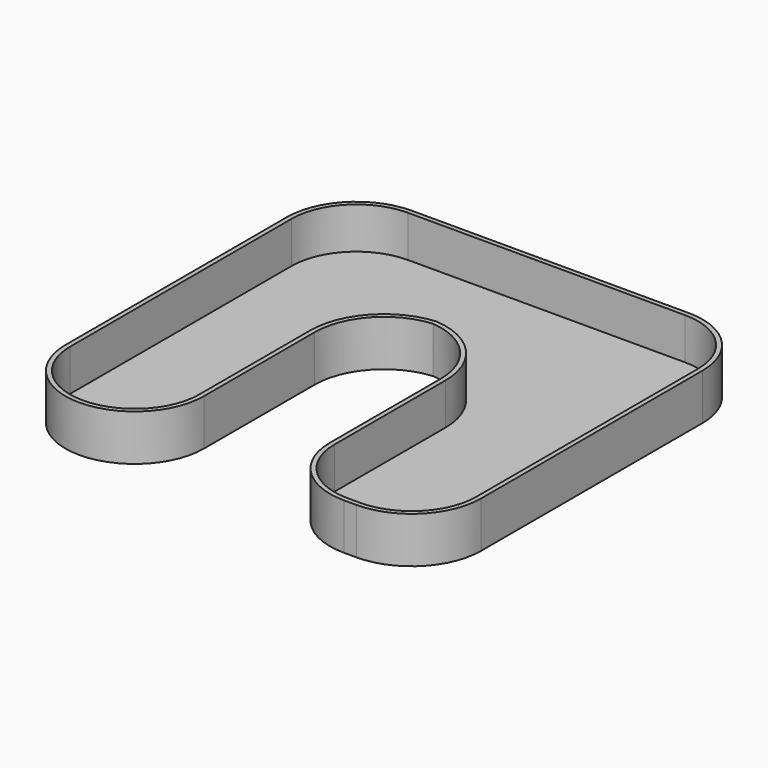
from build123d import *

# Parameters (mm, degrees)
F1_DEPTH    = 10
F2_T1_DEPTH = 10
F2_T3_DEPTH = 85
F3_T        = -1


# Not quite as in the source:
# - a fillet or chamfer that OpenCascade refuses, or shapes differently, is made with other operations: its cross-section is extruded or revolved along the edge and cut away or added


with BuildPart() as f1:
    # F0 (on Top) → F1 (new body)
    with BuildSketch(Plane.XY):
        Polygon((0, 90), (0, 0), (30, 0), (30, 60), (57.2968044168, 60), (57.2968044168, 0), (90, 0), (90, 90), align=None)
    extrude(amount=F1_DEPTH)

    # F2: fillet of radius 15 on 8 edges, made by hand

    # F2_s2 → F2_t1 (join)
    with BuildSketch(Plane.XY):
        with BuildLine():
            ThreePointArc((42.2968044168, 60), (52.9034061346, 55.6066017178), (57.2968044168, 45))
            Line((57.2968044168, 45), (57.2968044168, 60))
            Line((57.2968044168, 60), (42.2968044168, 60))
        make_face()
        with BuildLine():
            ThreePointArc((30, 45), (34.3933982822, 55.6066017178), (45, 60))
            Line((45, 60), (30, 60))
            Line((30, 60), (30, 45))
        make_face()
    extrude(amount=F2_T1_DEPTH)

    # F2_s4 → F2_t3 (cut)
    with BuildSketch(Plane.XY.offset(-37.5)):
        with BuildLine():
            ThreePointArc((75, 90), (85.6066017178, 85.6066017178), (90, 75))
            Line((90, 75), (90, 90))
            Line((90, 90), (75, 90))
        make_face()
        with BuildLine():
            ThreePointArc((90, 15), (85.6066017178, 4.3933982822), (75, 0))
            Line((75, 0), (90, 0))
            Line((90, 0), (90, 15))
        make_face()
        with BuildLine():
            ThreePointArc((15, 0), (25.6066017178, 4.3933982822), (30, 15))
            Line((30, 15), (30, 0))
            Line((30, 0), (15, 0))
        make_face()
        with BuildLine():
            ThreePointArc((57.2968044168, 15), (61.690202699, 4.3933982822), (72.2968044168, 0))
            Line((72.2968044168, 0), (57.2968044168, 0))
            Line((57.2968044168, 0), (57.2968044168, 15))
        make_face()
        with BuildLine():
            ThreePointArc((0, 15), (4.3933982822, 4.3933982822), (15, 0))
            Line((15, 0), (0, 0))
            Line((0, 0), (0, 15))
        make_face()
        with BuildLine():
            ThreePointArc((0, 75), (4.3933982822, 85.6066017178), (15, 90))
            Line((15, 90), (0, 90))
            Line((0, 90), (0, 75))
        make_face()
    extrude(amount=F2_T3_DEPTH, mode=Mode.SUBTRACT)

    # F3
    f3_openings = [f1.faces().sort_by_distance(p)[0] for p in [
        (5.293398, 84.706602, 10),
    ]]
    offset(amount=F3_T, openings=f3_openings, kind=Kind.INTERSECTION)


solid = f1.part
